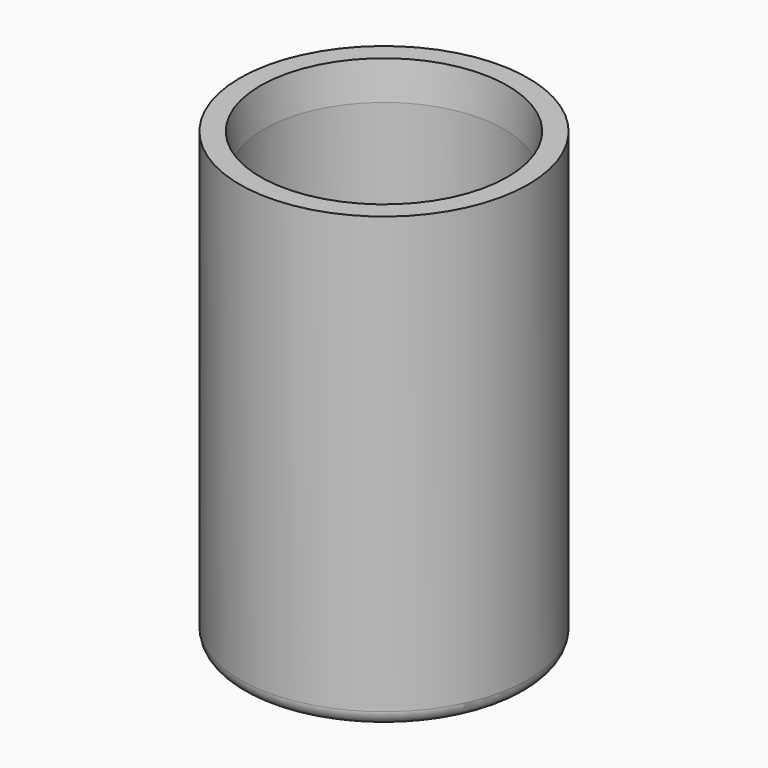
from build123d import *

# Parameters (mm, degrees)
F0_R     = 19.5140017551
F0_R_2   = 16.2285581311
F1_DEPTH = 2
F2_DEPTH = 59
F4_SIZE2 = 0.5
F4_SIZE  = 5


# Not quite as in the source:
# - a fillet or chamfer that OpenCascade refuses, or shapes differently, is made with other operations: its cross-section is extruded or revolved along the edge and cut away or added


with BuildPart() as f1:
    # F0 (on Top) → F1 (new body)
    with BuildSketch(Plane.XY):
        Circle(F0_R)
        Circle(F0_R_2, mode=Mode.SUBTRACT)
        Circle(F0_R_2)
    extrude(amount=-F1_DEPTH)

    # F0 (on Top) → F2 (join)
    with BuildSketch(Plane.XY):
        Circle(F0_R)
        Circle(F0_R_2, mode=Mode.SUBTRACT)
    extrude(amount=F2_DEPTH)

    # F3: fillet of radius 2 on 2 edges, made by hand

    # F3_s1 → F3_t2 (revolve, cut)
    with BuildSketch(Plane.XZ):
        with BuildLine():
            ThreePointArc((19.5140017551, 0), (18.9282153175, -1.4142135624), (17.5140017551, -2))
            Line((17.5140017551, -2), (19.5140017551, -2))
            Line((19.5140017551, -2), (19.5140017551, 0))
        make_face()
    revolve(axis=Axis((0, 0, -2), (0, 0, 1)), mode=Mode.SUBTRACT)

    # F3_s3 → F3_t4 (revolve)
    with BuildSketch(Plane.XZ):
        with BuildLine():
            ThreePointArc((16.2285581311, 2), (15.6427716934, 0.5857864376), (14.2285581311, 0))
            Line((14.2285581311, 0), (16.2285581311, 0))
            Line((16.2285581311, 0), (16.2285581311, 2))
        make_face()
    revolve(axis=Axis((0, 0, 0), (0, 0, 1)))

    # F4
    f4_edges = [f1.edges().sort_by_distance(p)[0] for p in [
        (-16.228558, 0, 59),
    ]]
    f4_side = f1.faces().sort_by_distance((-16.228558, 0, 30.5))[0]
    chamfer(f4_edges, length=F4_SIZE, length2=F4_SIZE2, reference=f4_side)


solid = f1.part
